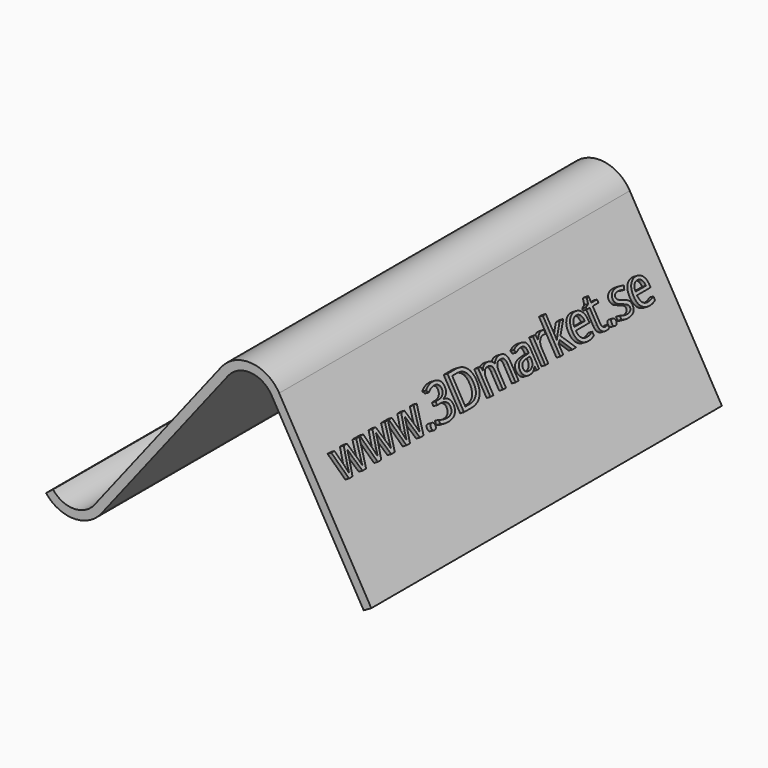
from build123d import *

# Parameters (mm, degrees)
F1_DEPTH     = 100
F2_TEXT_SIZE = 10.5257387205
F3_DEPTH     = 1


# Not quite as in the source:
# - Text() gives the source's letters only with a copy of the font that has no kerning and outlines rounded to 1/6400 em; it was checked with that copy


with BuildPart() as f1:
    # F0 (on Front) → F1 (new body)
    with BuildSketch(Plane.XZ):
        with BuildLine():
            ThreePointArc((-46.2603383651, 0), (-39.9537411232, -3.0779240937), (-33.6471438812, 0))
            Line((-33.6471438812, 0), (-4.7299479315, 37.0512587965))
            ThreePointArc((-4.7299479315, 37.0512587965), (0.4154860789, 39.345298856), (5.1946216651, 36.3623516559))
            Line((5.1946216651, 36.3623516559), (26.2131701891, 0))
            Line((26.2131701891, 0), (27.9447107441, 1.000883263))
            Line((27.9447107441, 1.000883263), (6.9261622202, 37.3632349189))
            ThreePointArc((6.9261622202, 37.3632349189), (0.5539814386, 41.3404978524), (-6.306597242, 38.2817777731))
            Line((-6.306597242, 38.2817777731), (-35.2237931917, 1.2305189766))
            ThreePointArc((-35.2237931917, 1.2305189766), (-39.9537411232, -1.0779240937), (-44.6836890546, 1.2305189766))
            Line((-44.6836890546, 1.2305189766), (-46.2603383651, 0))
        make_face()
    extrude(amount=F1_DEPTH)

    # F2 (on face) → F3 (join)
    with BuildSketch(Plane(origin=(21.379836522, 0, 12.3581977212), x_dir=(0, 1, 0), z_dir=(0.8657702775, 0, 0.5004416315))):
        with Locations((-95, 9.3718390372)):
            Text('www.3Dmarket.se', F2_TEXT_SIZE, font='Open Sans', text_align=(TextAlign.LEFT, TextAlign.BOTTOM))
    extrude(amount=F3_DEPTH)


solid = f1.part
